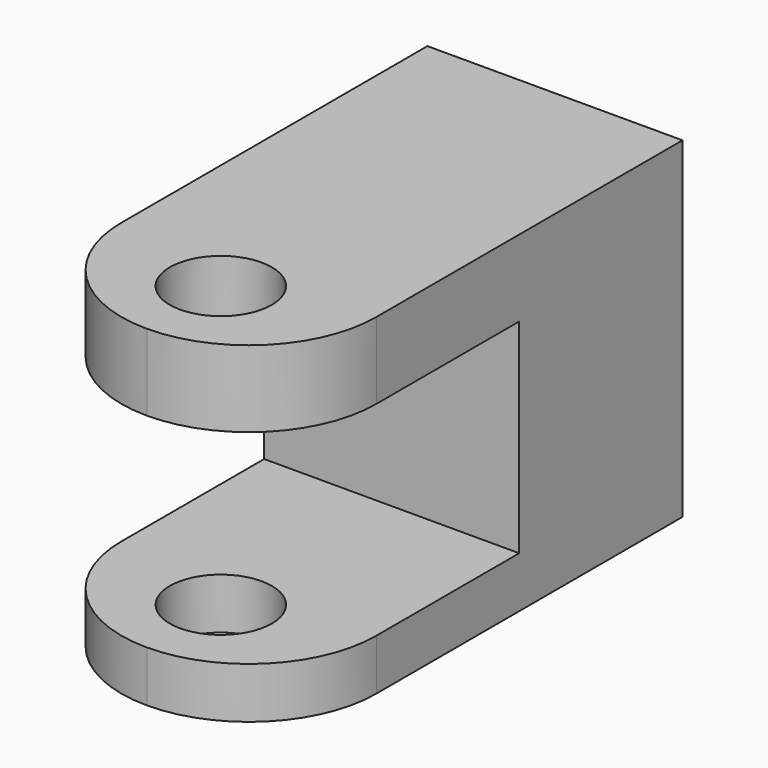
from build123d import *

# Parameters (mm, degrees)
F0_W     = 50
F0_H     = 65
F1_DEPTH = 40
F2_W     = 50
F2_H     = 15
F3_DEPTH = 60
F4_W     = 50
F4_H     = 10
F5_DEPTH = 60
F6_R     = 24.99999
F7_R     = 10
F8_DEPTH = 92.4


# Not quite as in the source:
# - a fillet or chamfer is up to 0.001 mm smaller than in the source, because OpenCascade refuses the exact size


with BuildPart() as f1:
    # F0 (on Front) → F1 (new body)
    with BuildSketch(Plane.XZ):
        with Locations((1.4840979129, -5.1116640333)):
            Rectangle(F0_W, F0_H)
    extrude(amount=F1_DEPTH)

    # F2 (on face) → F3 (join)
    with BuildSketch(Plane.XZ.offset(40)):
        with Locations((1.4840979129, 19.8883359667)):
            Rectangle(F2_W, F2_H)
    extrude(amount=F3_DEPTH)

    # F4 (on face) → F5 (join)
    with BuildSketch(Plane.XZ.offset(40)):
        with Locations((1.4840979129, -32.6116640333)):
            Rectangle(F4_W, F4_H)
    extrude(amount=F5_DEPTH)

    # F6 (radius 25 in the source; OpenCascade refuses exactly that, so slightly less here)
    f6_edges = [f1.edges().sort_by_distance(p)[0] for p in [
        (-23.515902, -100, -32.611664),
        (-23.515902, -100, 19.888336),
        (26.484098, -100, 19.888336),
        (26.484098, -100, -32.611664),
    ]]
    fillet(f6_edges, radius=F6_R)

    # F7 (on face) → F8 (cut)
    with BuildSketch(Plane.XY.offset(27.3883359667)):
        with Locations((1.4840979129, -81.8661674857)):
            Circle(F7_R)
    extrude(amount=-F8_DEPTH, mode=Mode.SUBTRACT)


solid = f1.part
